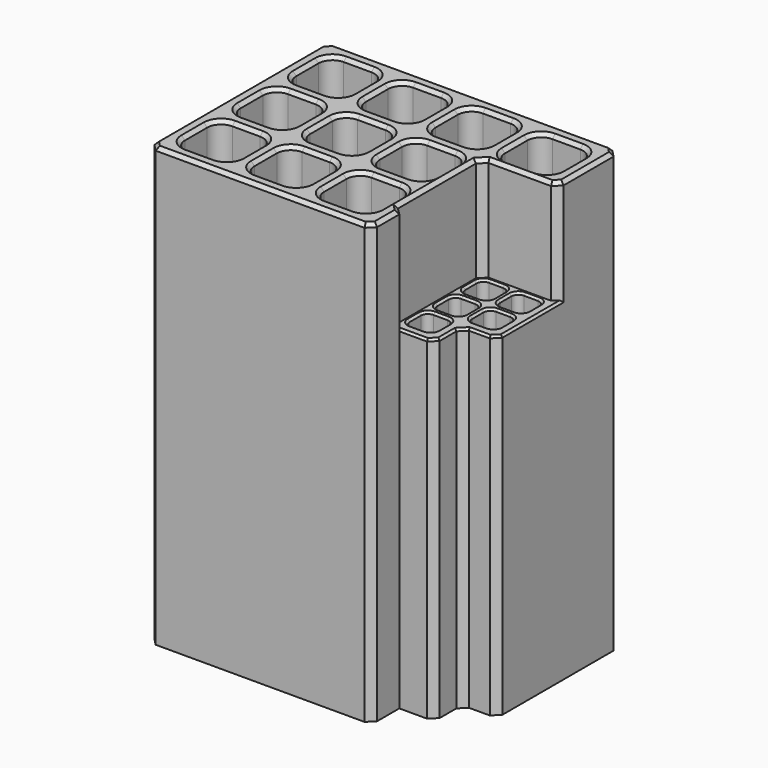
from build123d import *

# Parameters (mm, degrees)
F0_W     = 10
F0_H     = 10
F0_W_2   = 8
F0_H_2   = 8
F0_W_3   = 5.0117206536
F0_H_3   = 5
F0_W_4   = 4
F0_H_4   = 3.9906454055
F0_H_5   = 4
F0_H_6   = 1
F1_DEPTH = 3
F2_DEPTH = 60
F3_DEPTH = 45
F4_SIZE  = 1
F5_R     = 2
F6_R     = 1
F7_SIZE  = 1
F8_SIZE  = 0.49999
F9_SIZE  = 0.3


# Not quite as in the source:
# - a fillet or chamfer is up to 0.001 mm smaller than in the source, because OpenCascade refuses the exact size


with BuildPart() as f1:
    # F0 (on Top) → F1 (new body)
    with BuildSketch(Plane.XY):
        Polygon((-43.5472432673, 20), (-43.5472432673, 30), (-33.5472432673, 30), (-23.5472432673, 30), (-13.5472432673, 30), (-3.5472432673, 30), (-3.5472432673, 20), (-3.5355226137, 20), (-2.5472432673, 20.9882793464), (-2.5472432673, 31), (-3.5472432673, 31), (-44.5472432673, 31), (-44.5472432673, 30), (-44.5472432673, 0), (-44.5472432673, -1), (-13.5472432673, -1), (-12.5472432673, -1), (-12.5472432673, 4), (-13.5472432673, 5), (-13.5472432673, 0), (-23.5472432673, 0), (-33.5472432673, 0), (-43.5472432673, 0), (-43.5472432673, 10), align=None)
        with Locations((-38.5472432673, 25)):
            Rectangle(F0_W, F0_H)
        with Locations((-38.5472432673, 25)):
            Rectangle(F0_W_2, F0_H_2, mode=Mode.SUBTRACT)
        with Locations((-28.5472432673, 25)):
            Rectangle(F0_W, F0_H)
        with Locations((-28.5472432673, 25)):
            Rectangle(F0_W_2, F0_H_2, mode=Mode.SUBTRACT)
        with Locations((-38.5472432673, 15)):
            Rectangle(F0_W, F0_H)
        with Locations((-38.5472432673, 15)):
            Rectangle(F0_W_2, F0_H_2, mode=Mode.SUBTRACT)
        with Locations((-28.5472432673, 15)):
            Rectangle(F0_W, F0_H)
        with Locations((-28.5472432673, 15)):
            Rectangle(F0_W_2, F0_H_2, mode=Mode.SUBTRACT)
        with Locations((-38.5472432673, 5)):
            Rectangle(F0_W, F0_H)
        with Locations((-38.5472432673, 5)):
            Rectangle(F0_W_2, F0_H_2, mode=Mode.SUBTRACT)
        with Locations((-28.5472432673, 5)):
            Rectangle(F0_W, F0_H)
        with Locations((-28.5472432673, 5)):
            Rectangle(F0_W_2, F0_H_2, mode=Mode.SUBTRACT)
        Polygon((-13.5472432673, 10), (-23.5472432673, 10), (-23.5472432673, 0), (-13.5472432673, 0), (-13.5472432673, 5), (-13.5472432673, 6), align=None)
        with Locations((-18.5472432673, 5)):
            Rectangle(F0_W_2, F0_H_2, mode=Mode.SUBTRACT)
        Polygon((-13.5472432673, 20), (-23.5472432673, 20), (-23.5472432673, 10), (-13.5472432673, 10), (-13.5472432673, 12), (-13.5472432673, 15), (-13.5472432673, 18), align=None)
        with Locations((-18.5472432673, 15)):
            Rectangle(F0_W_2, F0_H_2, mode=Mode.SUBTRACT)
        with Locations((-18.5472432673, 25)):
            Rectangle(F0_W, F0_H)
        with Locations((-18.5472432673, 25)):
            Rectangle(F0_W_2, F0_H_2, mode=Mode.SUBTRACT)
        Polygon((-3.5472432673, 30), (-13.5472432673, 30), (-13.5472432673, 20), (-8.5472432673, 20), (-3.5472432673, 20), align=None)
        with Locations((-8.5472432673, 25)):
            Rectangle(F0_W_2, F0_H_2, mode=Mode.SUBTRACT)
        with Locations((-8.5472432673, 25)):
            Rectangle(F0_W_2, F0_H_2)
        with Locations((-28.5472432673, 15)):
            Rectangle(F0_W_2, F0_H_2)
        with Locations((-38.5472432673, 15)):
            Rectangle(F0_W_2, F0_H_2)
        with Locations((-38.5472432673, 5)):
            Rectangle(F0_W_2, F0_H_2)
        with Locations((-28.5472432673, 5)):
            Rectangle(F0_W_2, F0_H_2)
        with Locations((-18.5472432673, 5)):
            Rectangle(F0_W_2, F0_H_2)
        with Locations((-18.5472432673, 15)):
            Rectangle(F0_W_2, F0_H_2)
        with Locations((-18.5472432673, 25)):
            Rectangle(F0_W_2, F0_H_2)
        with Locations((-28.5472432673, 25)):
            Rectangle(F0_W_2, F0_H_2)
        with Locations((-38.5472432673, 25)):
            Rectangle(F0_W_2, F0_H_2)
        with Locations((-6.0413829405, 12.5)):
            Rectangle(F0_W_3, F0_H_3)
        with Locations((-6.0413829405, 12.5)):
            Rectangle(F0_W_4, F0_H_4, mode=Mode.SUBTRACT)
        Polygon((-3.5472432673, 20), (-8.5472432673, 20), (-8.5472432673, 15), (-3.5355226137, 15), (-3.5355226137, 20), align=None)
        with Locations((-6.0413829405, 17.5)):
            Rectangle(F0_W_4, F0_H_4, mode=Mode.SUBTRACT)
        Polygon((-8.5472432673, 10), (-13.5472432673, 10), (-13.5472432673, 6), (-13.5472432673, 5), (-12.5472432673, 5), (-8.5472432673, 5), (-8.5472432673, 9), align=None)
        with Locations((-11.0472432673, 7.5)):
            Rectangle(F0_W_4, F0_H_5, mode=Mode.SUBTRACT)
        Polygon((-8.5472432673, 20), (-13.5472432673, 20), (-13.5472432673, 18), (-13.5472432673, 15), (-8.5472432673, 15), align=None)
        with Locations((-11.0472432673, 17.5)):
            Rectangle(F0_W_4, F0_H_5, mode=Mode.SUBTRACT)
        Polygon((-13.5472432673, 12), (-13.5472432673, 10), (-8.5472432673, 10), (-8.5472432673, 15), (-13.5472432673, 15), align=None)
        with Locations((-11.0472432673, 12.5)):
            Rectangle(F0_W_4, F0_H_5, mode=Mode.SUBTRACT)
        with Locations((-11.0472432673, 7.5)):
            Rectangle(F0_W_4, F0_H_5)
        with Locations((-11.0472432673, 12.5)):
            Rectangle(F0_W_4, F0_H_5)
        with Locations((-11.0472432673, 17.5)):
            Rectangle(F0_W_4, F0_H_5)
        with Locations((-6.0413829405, 12.5)):
            Rectangle(F0_W_4, F0_H_4)
        with Locations((-6.0413829405, 17.5)):
            Rectangle(F0_W_4, F0_H_4)
        Polygon((-3.5355226137, 10), (-8.5472432673, 10), (-8.5472432673, 9), (-7.5472432673, 9), (-2.5472432673, 9), (-2.5472432673, 10), (-2.5472432673, 20), (-3.5355226137, 20), (-3.5355226137, 15), align=None)
        Polygon((-7.5472432673, 9), (-8.5472432673, 9), (-8.5472432673, 5), (-8.5472432673, 4), (-7.5472432673, 4), align=None)
        with Locations((-10.5472432673, 4.5)):
            Rectangle(F0_W_4, F0_H_6)
        Polygon((-12.5472432673, 5), (-13.5472432673, 5), (-12.5472432673, 4), align=None)
        Polygon((-2.5472432673, 20.9882793464), (-3.5355226137, 20), (-2.5472432673, 20), align=None)
    extrude(amount=-F1_DEPTH)

    # F0 (on Top) → F2 (join)
    with BuildSketch(Plane.XY):
        Polygon((-43.5472432673, 20), (-43.5472432673, 30), (-33.5472432673, 30), (-23.5472432673, 30), (-13.5472432673, 30), (-3.5472432673, 30), (-3.5472432673, 20), (-3.5355226137, 20), (-2.5472432673, 20.9882793464), (-2.5472432673, 31), (-3.5472432673, 31), (-44.5472432673, 31), (-44.5472432673, 30), (-44.5472432673, 0), (-44.5472432673, -1), (-13.5472432673, -1), (-12.5472432673, -1), (-12.5472432673, 4), (-13.5472432673, 5), (-13.5472432673, 0), (-23.5472432673, 0), (-33.5472432673, 0), (-43.5472432673, 0), (-43.5472432673, 10), align=None)
        with Locations((-38.5472432673, 25)):
            Rectangle(F0_W, F0_H)
        with Locations((-38.5472432673, 25)):
            Rectangle(F0_W_2, F0_H_2, mode=Mode.SUBTRACT)
        with Locations((-28.5472432673, 25)):
            Rectangle(F0_W, F0_H)
        with Locations((-28.5472432673, 25)):
            Rectangle(F0_W_2, F0_H_2, mode=Mode.SUBTRACT)
        with Locations((-38.5472432673, 15)):
            Rectangle(F0_W, F0_H)
        with Locations((-38.5472432673, 15)):
            Rectangle(F0_W_2, F0_H_2, mode=Mode.SUBTRACT)
        with Locations((-28.5472432673, 15)):
            Rectangle(F0_W, F0_H)
        with Locations((-28.5472432673, 15)):
            Rectangle(F0_W_2, F0_H_2, mode=Mode.SUBTRACT)
        with Locations((-38.5472432673, 5)):
            Rectangle(F0_W, F0_H)
        with Locations((-38.5472432673, 5)):
            Rectangle(F0_W_2, F0_H_2, mode=Mode.SUBTRACT)
        with Locations((-28.5472432673, 5)):
            Rectangle(F0_W, F0_H)
        with Locations((-28.5472432673, 5)):
            Rectangle(F0_W_2, F0_H_2, mode=Mode.SUBTRACT)
        Polygon((-13.5472432673, 10), (-23.5472432673, 10), (-23.5472432673, 0), (-13.5472432673, 0), (-13.5472432673, 5), (-13.5472432673, 6), align=None)
        with Locations((-18.5472432673, 5)):
            Rectangle(F0_W_2, F0_H_2, mode=Mode.SUBTRACT)
        Polygon((-13.5472432673, 20), (-23.5472432673, 20), (-23.5472432673, 10), (-13.5472432673, 10), (-13.5472432673, 12), (-13.5472432673, 15), (-13.5472432673, 18), align=None)
        with Locations((-18.5472432673, 15)):
            Rectangle(F0_W_2, F0_H_2, mode=Mode.SUBTRACT)
        with Locations((-18.5472432673, 25)):
            Rectangle(F0_W, F0_H)
        with Locations((-18.5472432673, 25)):
            Rectangle(F0_W_2, F0_H_2, mode=Mode.SUBTRACT)
        Polygon((-3.5472432673, 30), (-13.5472432673, 30), (-13.5472432673, 20), (-8.5472432673, 20), (-3.5472432673, 20), align=None)
        with Locations((-8.5472432673, 25)):
            Rectangle(F0_W_2, F0_H_2, mode=Mode.SUBTRACT)
    extrude(amount=F2_DEPTH)

    # F0 (on Top) → F3 (join)
    with BuildSketch(Plane.XY):
        Polygon((-8.5472432673, 20), (-13.5472432673, 20), (-13.5472432673, 18), (-13.5472432673, 15), (-8.5472432673, 15), align=None)
        with Locations((-11.0472432673, 17.5)):
            Rectangle(F0_W_4, F0_H_5, mode=Mode.SUBTRACT)
        Polygon((-13.5472432673, 12), (-13.5472432673, 10), (-8.5472432673, 10), (-8.5472432673, 15), (-13.5472432673, 15), align=None)
        with Locations((-11.0472432673, 12.5)):
            Rectangle(F0_W_4, F0_H_5, mode=Mode.SUBTRACT)
        Polygon((-8.5472432673, 10), (-13.5472432673, 10), (-13.5472432673, 6), (-13.5472432673, 5), (-12.5472432673, 5), (-8.5472432673, 5), (-8.5472432673, 9), align=None)
        with Locations((-11.0472432673, 7.5)):
            Rectangle(F0_W_4, F0_H_5, mode=Mode.SUBTRACT)
        with Locations((-6.0413829405, 12.5)):
            Rectangle(F0_W_3, F0_H_3)
        with Locations((-6.0413829405, 12.5)):
            Rectangle(F0_W_4, F0_H_4, mode=Mode.SUBTRACT)
        Polygon((-3.5472432673, 20), (-8.5472432673, 20), (-8.5472432673, 15), (-3.5355226137, 15), (-3.5355226137, 20), align=None)
        with Locations((-6.0413829405, 17.5)):
            Rectangle(F0_W_4, F0_H_4, mode=Mode.SUBTRACT)
        Polygon((-3.5355226137, 10), (-8.5472432673, 10), (-8.5472432673, 9), (-7.5472432673, 9), (-2.5472432673, 9), (-2.5472432673, 10), (-2.5472432673, 20), (-3.5355226137, 20), (-3.5355226137, 15), align=None)
        Polygon((-7.5472432673, 9), (-8.5472432673, 9), (-8.5472432673, 5), (-8.5472432673, 4), (-7.5472432673, 4), align=None)
        with Locations((-10.5472432673, 4.5)):
            Rectangle(F0_W_4, F0_H_6)
        Polygon((-12.5472432673, 5), (-13.5472432673, 5), (-12.5472432673, 4), align=None)
        Polygon((-2.5472432673, 20.9882793464), (-3.5355226137, 20), (-2.5472432673, 20), align=None)
    extrude(amount=F3_DEPTH)

    # F4
    f4_edges = [f1.edges().sort_by_distance(p)[0] for p in [
        (-2.547243, 31, 28.5),
        (-44.547243, 31, 28.5),
        (-44.547243, -1, 28.5),
        (-12.547243, -1, 28.5),
        (-7.547243, 4, 21),
        (-2.547243, 9, 21),
        (-7.547243, 9, 21),
    ]]
    chamfer(f4_edges, length=F4_SIZE)

    # F5
    f5_edges = [f1.edges().sort_by_distance(p)[0] for p in [
        (-42.547243, 29, 30),
        (-42.547243, 19, 30),
        (-42.547243, 9, 30),
        (-32.547243, 9, 30),
        (-32.547243, 19, 30),
        (-32.547243, 29, 30),
        (-22.547243, 29, 30),
        (-22.547243, 19, 30),
        (-22.547243, 9, 30),
        (-12.547243, 29, 30),
        (-4.547243, 29, 30),
        (-14.547243, 29, 30),
        (-24.547243, 29, 30),
        (-34.547243, 29, 30),
        (-24.547243, 19, 30),
        (-14.547243, 19, 30),
        (-14.547243, 9, 30),
        (-24.547243, 9, 30),
        (-34.547243, 9, 30),
        (-34.547243, 19, 30),
        (-34.547243, 11, 30),
        (-34.547243, 1, 30),
        (-34.547243, 21, 30),
        (-24.547243, 21, 30),
        (-24.547243, 11, 30),
        (-24.547243, 1, 30),
        (-14.547243, 1, 30),
        (-14.547243, 11, 30),
        (-14.547243, 21, 30),
        (-4.547243, 21, 30),
        (-22.547243, 1, 30),
        (-32.547243, 1, 30),
        (-42.547243, 1, 30),
        (-42.547243, 11, 30),
        (-32.547243, 11, 30),
        (-42.547243, 21, 30),
        (-32.547243, 21, 30),
        (-22.547243, 21, 30),
        (-12.547243, 21, 30),
        (-22.547243, 11, 30),
    ]]
    fillet(f5_edges, radius=F5_R)

    # F6
    f6_edges = [f1.edges().sort_by_distance(p)[0] for p in [
        (-13.047243, 19.5, 22.5),
        (-13.047243, 14.5, 22.5),
        (-13.047243, 9.5, 22.5),
        (-8.041383, 19.495323, 22.5),
        (-8.041383, 14.495323, 22.5),
        (-4.041383, 15.504677, 22.5),
        (-9.047243, 15.5, 22.5),
        (-4.041383, 10.504677, 22.5),
        (-9.047243, 10.5, 22.5),
        (-9.047243, 5.5, 22.5),
        (-9.047243, 9.5, 22.5),
        (-9.047243, 14.5, 22.5),
        (-9.047243, 19.5, 22.5),
        (-4.041383, 19.495323, 22.5),
        (-4.041383, 14.495323, 22.5),
        (-13.047243, 15.5, 22.5),
        (-8.041383, 15.504677, 22.5),
        (-8.041383, 10.504677, 22.5),
        (-13.047243, 10.5, 22.5),
        (-13.047243, 5.5, 22.5),
    ]]
    fillet(f6_edges, radius=F6_R)

    # F7
    f7_edges = [f1.edges().sort_by_distance(p)[0] for p in [
        (-13.547243, 20, 52.5),
    ]]
    chamfer(f7_edges, length=F7_SIZE)

    # F8 (size 0.5 in the source; OpenCascade refuses exactly that, so slightly less here)
    f8_edges = [f1.edges().sort_by_distance(p)[0] for p in [
        (-42.547243, 5, 60),
        (-42.547243, 15, 60),
        (-38.547243, 29, 60),
        (-28.547243, 29, 60),
        (-28.547243, 19, 0),
        (-30.547243, 19, 30),
        (-26.547243, 19, 30),
        (-28.547243, 19, 60),
        (-28.547243, 9, 0),
        (-30.547243, 9, 30),
        (-26.547243, 9, 30),
        (-28.547243, 9, 60),
        (-22.547243, 25, 60),
        (-18.547243, 19, 60),
        (-18.547243, 9, 60),
        (-12.547243, 25, 60),
        (-28.547243, -1, 60),
        (-13.047243, -0.5, 60),
        (-12.547243, 2, 60),
        (-13.547243, 12, 60),
        (-13.047243, 4.5, 60),
        (-13.047243, 19.5, 60),
        (-8.041383, 20, 60),
        (-3.041383, 20.49414, 60),
        (-2.547243, 25.49414, 60),
        (-44.547243, 15, 60),
        (-44.047243, -0.5, 60),
        (-3.047243, 30.5, 60),
        (-44.047243, 30.5, 60),
        (-23.547243, 31, 60),
    ]]
    chamfer(f8_edges, length=F8_SIZE)

    # F9
    f9_edges = [f1.edges().sort_by_distance(p)[0] for p in [
        (-13.047243, 17.5, 45),
        (-11.047243, 14.5, 45),
        (-11.047243, 9.5, 45),
        (-6.041383, 14.495323, 45),
        (-6.041383, 19.495323, 45),
        (-7.547243, 6.5, 45),
        (-7.047243, 8.5, 45),
        (-5.047243, 9, 45),
        (-2.547243, 15.49414, 45),
        (-3.047243, 9.5, 45),
        (-10.547243, 4, 45),
        (-8.047243, 4.5, 45),
    ]]
    chamfer(f9_edges, length=F9_SIZE)


solid = f1.part
